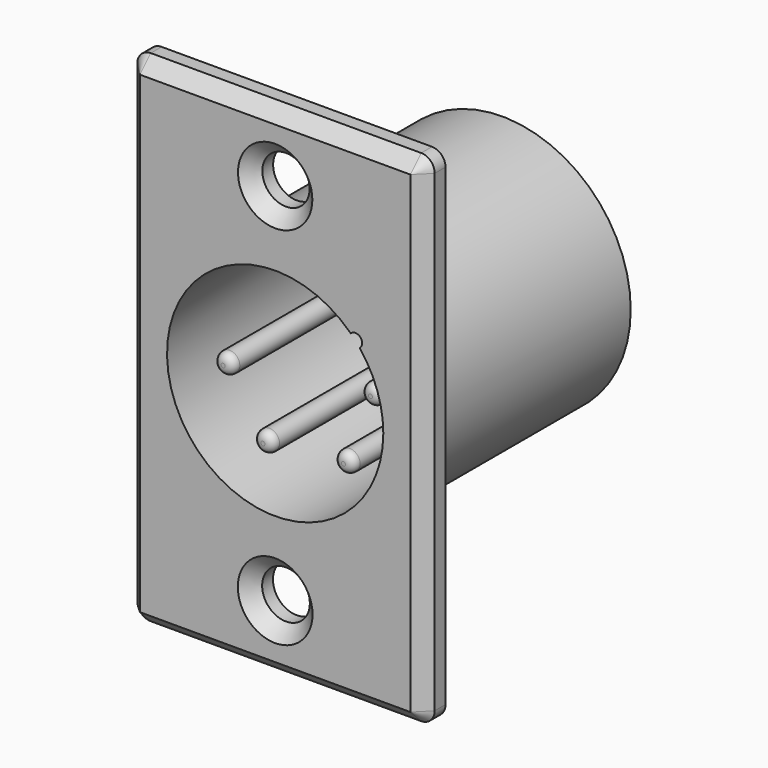
from build123d import *

# Parameters (mm, degrees)
F1_DEPTH  = 2
F2_R      = 9.5
F3_DEPTH  = 21
F5_DEPTH  = 16
F6_R      = 0.75
F7_DEPTH  = 14
F8_R      = 0.6
F9_R      = 1.765
F9_R_2    = 1.75
F10_DEPTH = 2
F11_SIZE  = 0.99999


# Not quite as in the source:
# - a fillet or chamfer is up to 0.001 mm smaller than in the source, because OpenCascade refuses the exact size


with BuildPart() as f1:
    # F0 (on Front) → F1 (new body)
    with BuildSketch(Plane.XZ):
        with BuildLine():
            Line((21, 0), (1, 0))
            ThreePointArc((1, 0), (0.2928932188, -0.2928932188), (0, -1))
            Line((0, -1), (0, -36))
            ThreePointArc((0, -36), (0.2928932188, -36.7071067812), (1, -37))
            Line((1, -37), (21, -37))
            ThreePointArc((21, -37), (21.7071067812, -36.7071067812), (22, -36))
            Line((22, -36), (22, -1))
            ThreePointArc((22, -1), (21.7071067812, -0.2928932188), (21, 0))
        make_face()
    extrude(amount=F1_DEPTH)

    # F2 (on face) → F3 (join)
    with BuildSketch(Plane.XZ.offset(2)):
        with Locations((11, -18.5)):
            Circle(F2_R)
    extrude(amount=-F3_DEPTH)

    # F4 (on face) → F5 (cut)
    with BuildSketch(Plane.XZ.offset(2)):
        with BuildLine():
            ThreePointArc((16.5855182065, -12.7726981601), (3.6282924077, -21.6077205753), (19, -18.5))
            ThreePointArc((19, -18.5), (18.5514473986, -15.8588558944), (17.2560894533, -13.5138848036))
            ThreePointArc((17.2560894533, -13.5138848036), (16.561616122, -13.4682581434), (16.5855182065, -12.7726981601))
        make_face()
        with BuildLine():
            ThreePointArc((16.5855182065, -12.7726981601), (16.561616122, -13.4682581434), (17.2560894533, -13.5138848036))
            ThreePointArc((17.2560894533, -13.5138848036), (16.9323905302, -13.1328086863), (16.5855182065, -12.7726981601))
        make_face()
        with BuildLine():
            ThreePointArc((16.5855182065, -12.7726981601), (16.9323905302, -13.1328086863), (17.2560894533, -13.5138848036))
            ThreePointArc((17.2560894533, -13.5138848036), (17.3861798324, -13.3427497952), (17.4323905302, -13.1328086863))
            ThreePointArc((17.4323905302, -13.1328086863), (17.128048188, -12.6726803554), (16.5855182065, -12.7726981601))
        make_face()
    extrude(amount=-F5_DEPTH, mode=Mode.SUBTRACT)

    # F6 (on face) → F7 (join)
    with BuildSketch(Plane.XZ.offset(-14)):
        with Locations((14.4535416495, -22.7805431986)):
            Circle(F6_R)
        with Locations((8.4928393267, -23.3953187188)):
            Circle(F6_R)
        with Locations((5.5545138952, -19.272451346)):
            Circle(F6_R)
        with Locations((16.4460298856, -17.7313918519)):
            Circle(F6_R)
    extrude(amount=F7_DEPTH)

    # F8
    f8_edges = [f1.edges().sort_by_distance(p)[0] for p in [
        (15.69603, 0, -17.731392),
        (13.703542, 0, -22.780543),
        (7.742839, 0, -23.395319),
        (4.804514, 0, -19.272451),
    ]]
    fillet(f8_edges, radius=F8_R)

    # F9 (on face) → F10 (cut, through all)
    with BuildSketch(Plane.XZ.offset(2)):
        with Locations((11, -32)):
            Circle(F9_R)
        with Locations((11, -5)):
            Circle(F9_R_2)
    extrude(amount=-F10_DEPTH, mode=Mode.SUBTRACT)

    # F11 (size 1 in the source; OpenCascade refuses exactly that, so slightly less here)
    f11_edges = [f1.edges().sort_by_distance(p)[0] for p in [
        (9.25, -2, -5),
        (9.235, -2, -32),
        (22, -2, -18.5),
        (11, -2, -37),
        (0, -2, -18.5),
        (11, -2, 0),
        (21.707107, -2, -0.292893),
        (0.292893, -2, -0.292893),
        (21.707107, -2, -36.707107),
        (0.292893, -2, -36.707107),
    ]]
    chamfer(f11_edges, length=F11_SIZE)


solid = f1.part
